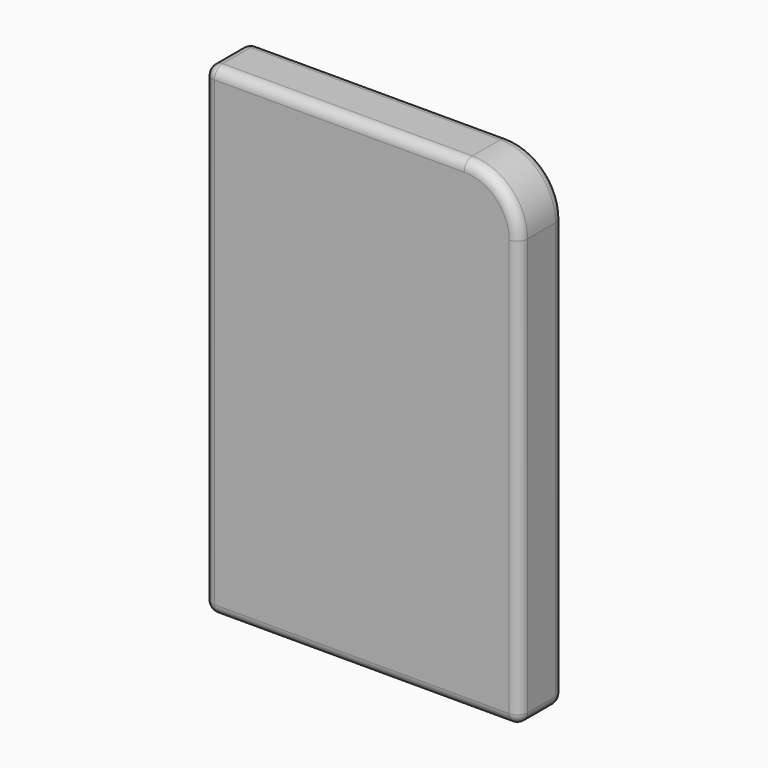
from build123d import *

# Parameters (mm, degrees)
F0_W         = 39.1473919153
F0_H         = 59.931833297
F1_DEPTH     = 6.87984
F2_R         = 6.858
F3_R         = 1.27
F4_T1_DEPTH  = 31.0193919153
F4_T3_DEPTH  = 36.6073919153
F4_T5_DEPTH  = 4.33984
F4_T7_DEPTH  = 51.803833297
F4_S11_W     = 1.27
F4_S11_H     = 1.27
F4_T12_DEPTH = 1.27
F4_S17_W     = 1.27
F4_S17_H     = 1.27
F4_T18_DEPTH = 1.27
F4_S23_W     = 1.27
F4_S23_H     = 1.27
F4_T24_DEPTH = 1.27
F4_S29_W     = 1.27
F4_S29_H     = 1.27
F4_T30_DEPTH = 1.27
F4_T34_ANGLE = 90
F4_T36_ANGLE = 90
F5_R         = 3
F6_DEPTH     = 8.18637
F7_R         = 1
F8_W         = 3.5
F8_H         = 3.25
F8_H_2       = 3.5
F8_W_2       = 3.25
F9_DEPTH     = 1.5
F10_R        = 0.5
F11_W        = 25.0252205878
F11_H        = 16.683479771
F12_DEPTH    = 0.74821
F14_DEPTH    = 0.76923
F16_DEPTH    = 0.6
F17_DEPTH    = 0.6
F18_T1_DEPTH = 2.831936667
F18_T3_DEPTH = 3.1
F18_T5_DEPTH = 3.4002586688
F19_T1_DEPTH = 3.1
F19_T3_DEPTH = 3.4002586688
F19_T5_DEPTH = 2.831936667
F20_R        = 1
F21_R        = 1
F22_R        = 1


# Not quite as in the source:
# - a fillet or chamfer that OpenCascade refuses, or shapes differently, is made with other operations: its cross-section is extruded or revolved along the edge and cut away or added


with BuildPart() as f1:
    # F0 (on Front) → F1 (new body)
    with BuildSketch(Plane.XZ):
        Rectangle(F0_W, F0_H)
    extrude(amount=-F1_DEPTH)

    # F2
    f2_edges = [f1.edges().sort_by_distance(p)[0] for p in [
        (19.573696, 3.43992, 29.965917),
    ]]
    fillet(f2_edges, radius=F2_R)

    # F3
    f3_edges = [f1.edges().sort_by_distance(p)[0] for p in [
        (-3.429, 6.87984, 29.965917),
        (-19.573696, 3.43992, 29.965917),
        (-19.573696, 3.43992, -29.965917),
        (-19.573696, 6.87984, 0),
        (-19.573696, 0, 0),
    ]]
    fillet(f3_edges, radius=F3_R)

    # F4: fillet of radius 1.27 on 3 edges, made by hand

    # F4_s2 → F4_t1 (cut)
    with BuildSketch(Plane.YZ.offset(-18.3036959577)):
        with BuildLine():
            ThreePointArc((1.27, 29.9659166485), (0.3719743879, 29.5939422606), (0, 28.6959166485))
            Line((0, 28.6959166485), (0, 29.9659166485))
            Line((0, 29.9659166485), (1.27, 29.9659166485))
        make_face()
    extrude(amount=F4_T1_DEPTH, mode=Mode.SUBTRACT)

    # F4_s4 → F4_t3 (cut)
    with BuildSketch(Plane.YZ.offset(-18.3036959577)):
        with BuildLine():
            ThreePointArc((5.60984, -29.9659166485), (6.5078656121, -29.5939422606), (6.87984, -28.6959166485))
            Line((6.87984, -28.6959166485), (6.87984, -29.9659166485))
            Line((6.87984, -29.9659166485), (5.60984, -29.9659166485))
        make_face()
        with BuildLine():
            ThreePointArc((0, -28.6959166485), (0.3719743879, -29.5939422606), (1.27, -29.9659166485))
            Line((1.27, -29.9659166485), (0, -29.9659166485))
            Line((0, -29.9659166485), (0, -28.6959166485))
        make_face()
    extrude(amount=F4_T3_DEPTH, mode=Mode.SUBTRACT)

    # F4_s6 → F4_t5 (cut)
    with BuildSketch(Plane.XZ.offset(-5.60984)):
        with BuildLine():
            ThreePointArc((18.3036959577, -29.9659166485), (19.2017215698, -29.5939422606), (19.5736959577, -28.6959166485))
            Line((19.5736959577, -28.6959166485), (19.5736959577, -29.9659166485))
            Line((19.5736959577, -29.9659166485), (18.3036959577, -29.9659166485))
        make_face()
    extrude(amount=F4_T5_DEPTH, mode=Mode.SUBTRACT)

    # F4_s8 → F4_t7 (cut)
    with BuildSketch(Plane.XY.offset(-28.6959166485)):
        with BuildLine():
            ThreePointArc((18.3036959577, 0), (19.2017215698, 0.3719743879), (19.5736959577, 1.27))
            Line((19.5736959577, 1.27), (19.5736959577, 0))
            Line((19.5736959577, 0), (18.3036959577, 0))
        make_face()
    extrude(amount=F4_T7_DEPTH, mode=Mode.SUBTRACT)


with BuildPart() as f4_tool10:
    # F4_s11 → F4_t12 (new body)
    with BuildSketch(Plane.XZ.offset(-1.27)):
        with Locations((-18.9386959577, -29.3309166485)):
            Rectangle(F4_S11_W, F4_S11_H)
    extrude(amount=F4_T12_DEPTH)

    # F4_s13 → F4_t14 (revolve, cut)
    with BuildSketch(Plane(origin=(-18.3036959577, 1.27, -28.6959166485), x_dir=(0.7071067812, 0, 0.7071067812), z_dir=(0.7071067812, 0, -0.7071067812))):
        with BuildLine():
            ThreePointArc((0, -1.27), (1.27, 0), (0, 1.27))
            Line((0, 1.27), (0, -1.27))
        make_face()
    revolve(axis=Axis((-18.3036959577, 1.27, -28.6959166485), (0, -1, 0)), mode=Mode.SUBTRACT)


with BuildPart() as f1_1:
    add(f1.part)

    # F4_t9: cut F4_tool10
    add(f4_tool10.part, mode=Mode.SUBTRACT)


with BuildPart() as f4_tool16:
    # F4_s17 → F4_t18 (new body)
    with BuildSketch(Plane.XY.offset(-28.6959166485)):
        with Locations((-18.9386959577, 6.24484)):
            Rectangle(F4_S17_W, F4_S17_H)
    extrude(amount=-F4_T18_DEPTH)

    # F4_s19 → F4_t20 (revolve, cut)
    with BuildSketch(Plane(origin=(-18.3036959577, 5.60984, -28.6959166485), x_dir=(0.7071067812, -0.7071067812, 0), z_dir=(0.7071067812, 0.7071067812, 0))):
        with BuildLine():
            ThreePointArc((0, -1.27), (1.27, 0), (0, 1.27))
            Line((0, 1.27), (0, -1.27))
        make_face()
    revolve(axis=Axis((-18.3036959577, 5.60984, -28.6959166485), (0, 0, -1)), mode=Mode.SUBTRACT)


with BuildPart() as f1_2:
    add(f1_1.part)

    # F4_t15: cut F4_tool16
    add(f4_tool16.part, mode=Mode.SUBTRACT)


with BuildPart() as f4_tool22:
    # F4_s23 → F4_t24 (new body)
    with BuildSketch(Plane.XY.offset(28.6959166485)):
        with Locations((-18.9386959577, 0.635)):
            Rectangle(F4_S23_W, F4_S23_H)
    extrude(amount=F4_T24_DEPTH)

    # F4_s25 → F4_t26 (revolve, cut)
    with BuildSketch(Plane(origin=(-18.3036959577, 1.27, 28.6959166485), x_dir=(0.7071067812, 0.7071067812, 0), z_dir=(0.7071067812, -0.7071067812, 0))):
        with BuildLine():
            ThreePointArc((0, -1.27), (1.27, 0), (0, 1.27))
            Line((0, 1.27), (0, -1.27))
        make_face()
    revolve(axis=Axis((-18.3036959577, 1.27, 28.6959166485), (0, 0, 1)), mode=Mode.SUBTRACT)


with BuildPart() as f1_3:
    add(f1_2.part)

    # F4_t21: cut F4_tool22
    add(f4_tool22.part, mode=Mode.SUBTRACT)


with BuildPart() as f4_tool28:
    # F4_s29 → F4_t30 (new body)
    with BuildSketch(Plane.XZ.offset(-1.27)):
        with Locations((18.9386959577, -29.3309166485)):
            Rectangle(F4_S29_W, F4_S29_H)
    extrude(amount=F4_T30_DEPTH)

    # F4_s31 → F4_t32 (revolve, cut)
    with BuildSketch(Plane(origin=(18.3036959577, 1.27, -28.6959166485), x_dir=(-0.7071067812, 0, 0.7071067812), z_dir=(0.7071067812, 0, 0.7071067812))):
        with BuildLine():
            ThreePointArc((0, -1.27), (1.27, 0), (0, 1.27))
            Line((0, 1.27), (0, -1.27))
        make_face()
    revolve(axis=Axis((18.3036959577, 1.27, -28.6959166485), (0, -1, 0)), mode=Mode.SUBTRACT)


with BuildPart() as f1_4:
    add(f1_3.part)

    # F4_t27: cut F4_tool28
    add(f4_tool28.part, mode=Mode.SUBTRACT)

    # F4_s33 → F4_t34 (revolve, cut)
    with BuildSketch(Plane.XZ.offset(-5.60984)):
        with BuildLine():
            ThreePointArc((18.3036959577, -29.9659166485), (19.2017215698, -29.5939422606), (19.5736959577, -28.6959166485))
            Line((19.5736959577, -28.6959166485), (19.5736959577, -29.9659166485))
            Line((19.5736959577, -29.9659166485), (18.3036959577, -29.9659166485))
        make_face()
    revolve(axis=Axis((18.3036959577, 5.60984, -29.9659166485), (0, 0, 1)), revolution_arc=F4_T34_ANGLE, mode=Mode.SUBTRACT)

    # F4_s35 → F4_t36 (revolve, cut)
    with BuildSketch(Plane.YZ.offset(12.7156959577)):
        with BuildLine():
            ThreePointArc((0, 28.6959166485), (0.3719743879, 29.5939422606), (1.27, 29.9659166485))
            Line((1.27, 29.9659166485), (0, 29.9659166485))
            Line((0, 29.9659166485), (0, 28.6959166485))
        make_face()
    revolve(axis=Axis((12.7156959577, 0, 23.1079166485), (0, 1, 0)), revolution_arc=F4_T36_ANGLE, mode=Mode.SUBTRACT)

    # F5 (on Front) → F6 (join)
    with BuildSketch(Plane.XZ):
        with Locations((13.5736959577, 5)):
            Circle(F5_R)
        with Locations((4.1767697498, 8.4202014333)):
            Circle(F5_R)
    extrude(amount=-F6_DEPTH)

    # F7
    f7_edges = [f1_4.edges().sort_by_distance(p)[0] for p in [
        (1.17677, 8.18637, 8.420201),
        (10.573696, 8.18637, 5),
    ]]
    fillet(f7_edges, radius=F7_R)

    # F8 (on face) → F9 (join)
    with BuildSketch(Plane(origin=(0, 6.87984, 0), x_dir=(-1, 0, 0), z_dir=(0, 1, 0))):
        with Locations((10.2288695052, 9.5590941198)):
            Rectangle(F8_W, F8_H)
        with Locations((10.2288695052, 6.1840941198)):
            Rectangle(F8_W, F8_H_2)
        with Locations((6.8538695052, 6.1840941198)):
            Rectangle(F8_W_2, F8_H_2)
        with Locations((13.6038695052, 6.1840941198)):
            Rectangle(F8_W_2, F8_H_2)
        with Locations((10.2288695052, 2.8090941198)):
            Rectangle(F8_W, F8_H)
    extrude(amount=F9_DEPTH)

    # F10
    f10_edges = [f1_4.edges().sort_by_distance(p)[0] for p in [
        (-8.47887, 8.37984, 9.559094),
        (-6.85387, 8.37984, 7.934094),
        (-5.22887, 8.37984, 6.184094),
        (-6.85387, 8.37984, 4.434094),
        (-8.47887, 8.37984, 2.809094),
        (-10.22887, 8.37984, 1.184094),
        (-11.97887, 8.37984, 2.809094),
        (-13.60387, 8.37984, 4.434094),
        (-15.22887, 8.37984, 6.184094),
        (-13.60387, 8.37984, 7.934094),
        (-11.97887, 8.37984, 9.559094),
        (-10.22887, 8.37984, 11.184094),
    ]]
    fillet(f10_edges, radius=F10_R)

    # F11 (on face) → F12 (cut)
    with BuildSketch(Plane(origin=(0, 6.87984, 0), x_dir=(-1, 0, 0), z_dir=(0, 1, 0))):
        with Locations((0, -13.0091430619)):
            Rectangle(F11_W, F11_H)
    extrude(amount=-F12_DEPTH, mode=Mode.SUBTRACT)

    # F13 (on face) → F14 (cut)
    with BuildSketch(Plane(origin=(0, 6.87984, 0), x_dir=(-1, 0, 0), z_dir=(0, 1, 0))):
        Polygon((-15.8662368542, 22.8707954266), (-16.3716748357, 22.3865099251), (-12.2206562519, 18.0541843698), (-11.7152182705, 18.5384698712), align=None)
        Polygon((-11.1337694753, 19.0879527843), (-10.6283314938, 19.5722382857), (-14.7793500776, 23.904563841), (-15.284788059, 23.4202783396), align=None)
        Polygon((-10.0468826986, 20.1217211988), (-9.5414447172, 20.6060067002), (-13.6924633009, 24.9383322555), (-14.1979012824, 24.4540467541), align=None)
        Polygon((-8.959995922, 21.1554896132), (-8.4545579406, 21.6397751147), (-12.6055765243, 25.97210067), (-13.1110145058, 25.4878151686), align=None)
        Polygon((-7.8731091454, 22.1892580277), (-7.3676711639, 22.6735435291), (-11.5186897477, 27.0058690845), (-12.0241277291, 26.521583583), align=None)
        Polygon((-6.7862223687, 23.2230264422), (-6.2807843873, 23.7073119436), (-10.431802971, 28.0396374989), (-10.9372409525, 27.5553519975), align=None)
    extrude(amount=-F14_DEPTH, mode=Mode.SUBTRACT)

    # F15 (on face) → F16 (join)
    with BuildSketch(Plane(origin=(0, 6.87984, 0), x_dir=(-1, 0, 0), z_dir=(0, 1, 0))):
        Polygon((4.9829966579, 15.9248658988), (5.6341970339, 14.6409766749), (12.4587174505, 17.180332914), (11.9598941685, 18.5209205872), align=None)
    extrude(amount=F16_DEPTH)

    # F15 (on face) → F17 (join)
    with BuildSketch(Plane(origin=(0, 6.87984, 0), x_dir=(-1, 0, 0), z_dir=(0, 1, 0))):
        Polygon((4.9829966579, 15.9248658988), (5.6341970339, 14.6409766749), (12.4587174505, 17.180332914), (11.9598941685, 18.5209205872), align=None)
        Polygon((-3.5166739851, 15.999692095), (-2.8654736091, 14.715802871), (3.9590468074, 17.2551591101), (3.4602235255, 18.5957467833), align=None)
    extrude(amount=F17_DEPTH)

    # F18: fillet of radius 1 on 4 edges, made by hand

    # F18_s2 → F18_t1 (cut)
    with BuildSketch(Plane.XZ.offset(-9.711776667)):
        with BuildLine():
            ThreePointArc((-5.2303506466, 15.4371893983), (-5.7581630774, 14.9581512114), (-6.4709249675, 14.9523172774))
            Line((-6.4709249675, 14.9523172774), (-5.6341970339, 14.6409766749))
            Line((-5.6341970339, 14.6409766749), (-5.2303506466, 15.4371893983))
        make_face()
    extrude(amount=F18_T1_DEPTH, mode=Mode.SUBTRACT)

    # F18_s4 → F18_t3 (cut)
    with BuildSketch(Plane.XZ.offset(-9.97984)):
        with BuildLine():
            ThreePointArc((-12.109983762, 18.1175547738), (-12.0820697907, 17.3526971087), (-11.5214955907, 16.8315992255))
            Line((-11.5214955907, 16.8315992255), (-12.4587174505, 17.180332914))
            Line((-12.4587174505, 17.180332914), (-12.109983762, 18.1175547738))
        make_face()
        with BuildLine():
            ThreePointArc((-11.0226723087, 18.1721868987), (-11.7875299738, 18.1442729274), (-12.308627857, 17.5836987274))
            Line((-12.308627857, 17.5836987274), (-11.9598941685, 18.5209205872))
            Line((-11.9598941685, 18.5209205872), (-11.0226723087, 18.1721868987))
        make_face()
    extrude(amount=F18_T3_DEPTH, mode=Mode.SUBTRACT)

    # F18_s6 → F18_t5 (cut)
    with BuildSketch(Plane.XZ.offset(-10.2800986688)):
        with BuildLine():
            ThreePointArc((-6.032782113, 16.3154837126), (-5.4501278756, 15.7422900544), (-5.489675169, 14.9259121139))
            Line((-5.489675169, 14.9259121139), (-4.9829966579, 15.9248658988))
            Line((-4.9829966579, 15.9248658988), (-6.032782113, 16.3154837126))
        make_face()
    extrude(amount=F18_T5_DEPTH, mode=Mode.SUBTRACT)

    # F19: fillet of radius 1 on 4 edges, made by hand

    # F19_s2 → F19_t1 (cut)
    with BuildSketch(Plane.XZ.offset(-9.97984)):
        with BuildLine():
            ThreePointArc((-3.808957214, 17.6585249235), (-3.2878593307, 18.2190991235), (-2.5230016657, 18.2470130948))
            Line((-2.5230016657, 18.2470130948), (-3.4602235255, 18.5957467833))
            Line((-3.4602235255, 18.5957467833), (-3.808957214, 17.6585249235))
        make_face()
        with BuildLine():
            ThreePointArc((-3.6103131189, 18.1923809699), (-3.5823991476, 17.4275233048), (-3.0218249476, 16.9064254216))
            Line((-3.0218249476, 16.9064254216), (-3.9590468074, 17.2551591101))
            Line((-3.9590468074, 17.2551591101), (-3.6103131189, 18.1923809699))
        make_face()
    extrude(amount=F19_T1_DEPTH, mode=Mode.SUBTRACT)

    # F19_s4 → F19_t3 (cut)
    with BuildSketch(Plane.XZ.offset(-10.2800986688)):
        with BuildLine():
            ThreePointArc((2.4668885301, 16.3903099087), (3.0495427674, 15.8171162505), (3.0099954741, 15.00073831))
            Line((3.0099954741, 15.00073831), (3.5166739851, 15.999692095))
            Line((3.5166739851, 15.999692095), (2.4668885301, 16.3903099087))
        make_face()
    extrude(amount=F19_T3_DEPTH, mode=Mode.SUBTRACT)

    # F19_s6 → F19_t5 (cut)
    with BuildSketch(Plane.XZ.offset(-9.711776667)):
        with BuildLine():
            ThreePointArc((2.0287456755, 15.0271434735), (2.7415075656, 15.0329774075), (3.2693199965, 15.5120155945))
            Line((3.2693199965, 15.5120155945), (2.8654736091, 14.715802871))
            Line((2.8654736091, 14.715802871), (2.0287456755, 15.0271434735))
        make_face()
    extrude(amount=F19_T5_DEPTH, mode=Mode.SUBTRACT)

    # F20
    f20_edges = [f1_4.edges().sort_by_distance(p)[0] for p in [
        (12.51261, 6.505735, -21.350883),
    ]]
    fillet(f20_edges, radius=F20_R)

    # F21
    f21_edges = [f1_4.edges().sort_by_distance(p)[0] for p in [
        (12.51261, 6.505735, -4.667403),
    ]]
    fillet(f21_edges, radius=F21_R)

    # F22
    f22_edges = [f1_4.edges().sort_by_distance(p)[0] for p in [
        (-12.51261, 6.505735, -4.667403),
        (-12.51261, 6.505735, -21.350883),
    ]]
    fillet(f22_edges, radius=F22_R)


solid = f1_4.part
